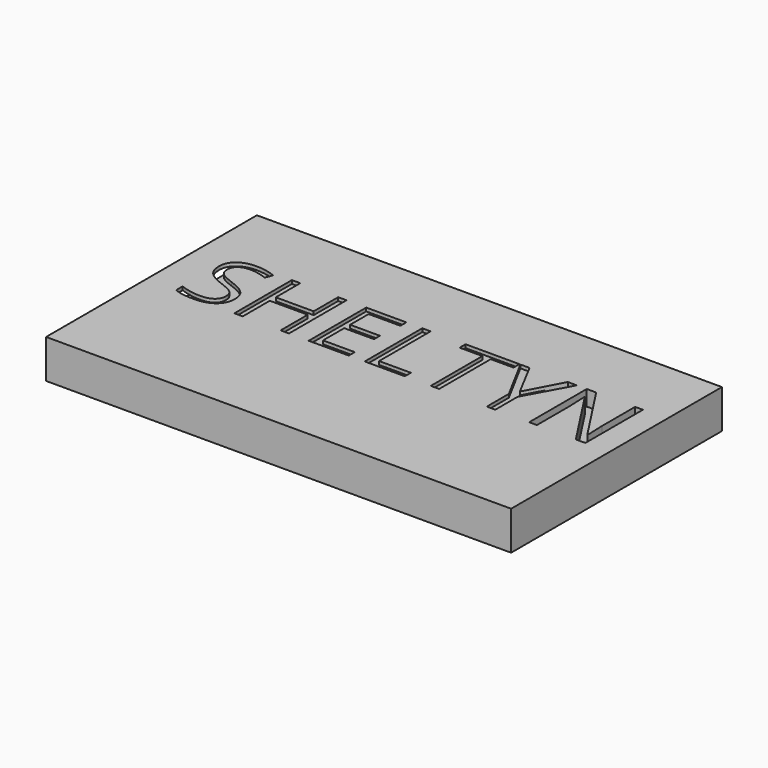
from build123d import *

# Parameters (mm, degrees)
F0_W          = 76.2
F0_H          = 43.18
F1_DEPTH      = 6.35
F2_W          = 41.8452303857
F2_H          = 5.2806600579
F3_DEPTH      = 58.42
F4_W          = 19.3852782249
F4_H          = 36.3931208849
F5_DEPTH      = 2.54
F6_W          = 1.0002194852
F6_H          = 5.2806600579
F7_DEPTH      = 2.54
F8_T1_DEPTH   = 5.2806600579
F9_W          = 3.2472847909
F9_H          = 5.2806600579
F10_DEPTH     = 1.27
F11_SIZE      = 1.26999
F12_T1_DEPTH  = 5.2806600579
F13_R         = 1.27
F14_TEXT_SIZE = 16.5100002454
F15_DEPTH     = 2.54


# Not quite as in the source:
# - a fillet or chamfer that OpenCascade refuses, or shapes differently, is made with other operations: its cross-section is extruded or revolved along the edge and cut away or added
# - a fillet or chamfer is up to 0.001 mm smaller than in the source, because OpenCascade refuses the exact size
# - Text() gives the source's letters only with a copy of the font that has no kerning and outlines rounded to 1/6400 em; it was checked with that copy


with BuildPart() as f1:
    # F0 (on Top) → F1 (new body)
    with BuildSketch(Plane.XY):
        with Locations((2.9745269567, 0.6024450838)):
            Rectangle(F0_W, F0_H)
    extrude(amount=F1_DEPTH)

    # F2 (on face) → F3 (cut)
    with BuildSketch(Plane(origin=(-35.1254730433, 0, 0), x_dir=(0, -1, 0), z_dir=(-1, 0, 0))):
        with Locations((-0.5776667967, 3.1501960184)):
            Rectangle(F2_W, F2_H)
    extrude(amount=-F3_DEPTH, mode=Mode.SUBTRACT)

    # F4 (on face) → F5 (cut)
    with BuildSketch(Plane(origin=(0, 0, 0), x_dir=(1, 0, 0), z_dir=(0, 0, -1))):
        with Locations((28.346400708, -0.1828800887)):
            Rectangle(F4_W, F4_H)
    extrude(amount=-F5_DEPTH, mode=Mode.SUBTRACT)

    # F6 (on face) → F7 (join)
    with BuildSketch(Plane.XZ.offset(-21.5002819896)):
        with Locations((-34.6253633007, 3.1501960184)):
            Rectangle(F6_W, F6_H)
    extrude(amount=F7_DEPTH)

    # F8: chamfer of 1.27 on 1 edges, made by hand

    # F8_s2 → F8_t1 (cut)
    with BuildSketch(Plane.XY.offset(0.5098659894)):
        Polygon((-35.3952535582, 18.9602819896), (-34.1252535582, 20.2302819896), (-34.1252535582, 18.9602819896), align=None)
    extrude(amount=F8_T1_DEPTH, mode=Mode.SUBTRACT)

    # F9 (on face) → F10 (join)
    with BuildSketch(Plane(origin=(0, -20.3449483961, 0), x_dir=(-1, 0, 0), z_dir=(0, 1, 0))):
        with Locations((33.5018306479, 3.1501960184)):
            Rectangle(F9_W, F9_H)
    extrude(amount=F10_DEPTH)

    # F11 (size 1.27 in the source; OpenCascade refuses exactly that, so slightly less here)
    f11_edges = [f1.edges().sort_by_distance(p)[0] for p in [
        (-31.878188, -19.074948, 3.150196),
    ]]
    chamfer(f11_edges, length=F11_SIZE)

    # F12: fillet of radius 1.27 on 1 edges, made by hand

    # F12_s2 → F12_t1 (cut)
    with BuildSketch(Plane.XY.offset(0.5098659894)):
        with BuildLine():
            ThreePointArc((-35.1254730433, 21.4712970877), (-34.8442908359, 20.6743407696), (-34.1252535582, 20.2302819896))
            Line((-34.1252535582, 20.2302819896), (-35.1254730433, 19.2300625045))
            Line((-35.1254730433, 19.2300625045), (-35.1254730433, 21.4712970877))
        make_face()
    extrude(amount=F12_T1_DEPTH, mode=Mode.SUBTRACT)

    # F13
    f13_edges = [f1.edges().sort_by_distance(p)[0] for p in [
        (-35.125473, -19.074948, 3.150196),
    ]]
    fillet(f13_edges, radius=F13_R)

    # F14 (on face) → F15 (cut)
    with BuildSketch(Plane.XY.offset(6.35)):
        with Locations((-31.0896020383, -0.8229594678)):
            Text('SHELTYN', F14_TEXT_SIZE, font='Open Sans', text_align=(TextAlign.LEFT, TextAlign.BOTTOM))
    extrude(amount=-F15_DEPTH, mode=Mode.SUBTRACT)


solid = f1.part
